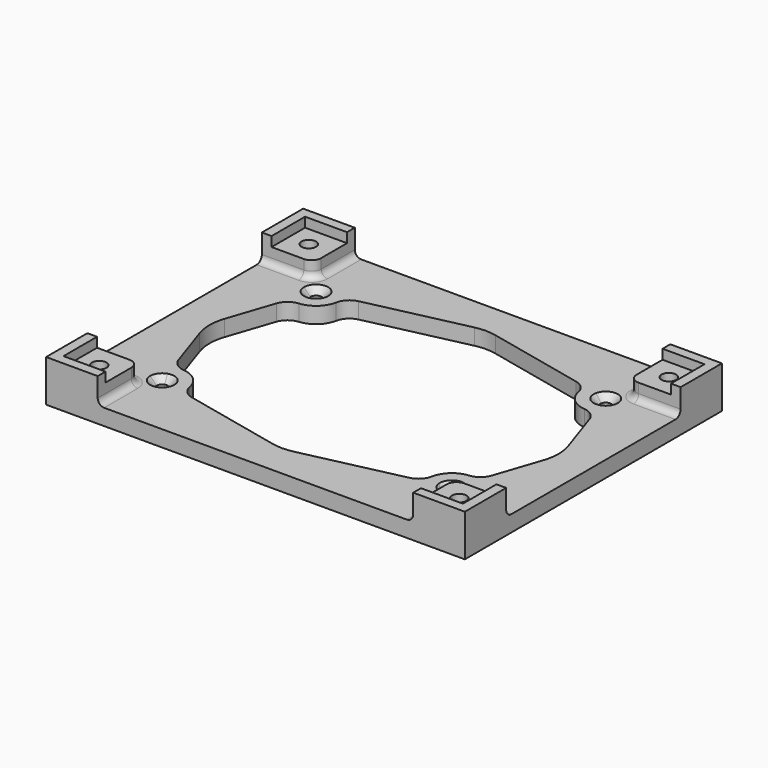
from build123d import *

# Parameters (mm, degrees)
F1_DEPTH = 5
F0_W     = 13
F0_H     = 13
F0_R     = 4
F0_R_2   = 2.25
F2_DEPTH = 10
F3_DEPTH = 13
F4_DEPTH = 6
F5_SIZE  = 2
F6_R     = 3
F7_R     = 2
F8_R     = 5
F11_R    = 15


with BuildPart() as f1:
    # F0 (on Top) → F1 (new body)
    with BuildSketch(Plane.XY):
        with BuildLine():
            ThreePointArc((43.1918518623, 30.1804338837), (45.0913645201, 31.5395055678), (46.65, 29.8))
            ThreePointArc((46.65, 29.8), (46.3207025236, 28.7781857608), (45.4567378977, 28.1409210648))
            Line((45.4567378977, 28.1409210648), (47.2860195617, 22.6896617063))
            Line((47.2860195617, 22.6896617063), (54.9, 0))
            Line((54.9, 0), (64.9, 0))
            Line((64.9, 0), (64.9, 33.8))
            Line((64.9, 33.8), (61.9, 33.8))
            Line((61.9, 33.8), (48.9, 33.8))
            Line((48.9, 33.8), (48.9, 46.8))
            Line((48.9, 46.8), (48.9, 49.8))
            Line((48.9, 49.8), (0, 49.8))
            Line((0, 49.8), (0, 39.8))
            Line((0, 39.8), (37.5793651244, 31.43043093))
            Line((37.5793651244, 31.43043093), (43.1918518623, 30.1804338837))
        make_face()
        with BuildLine():
            ThreePointArc((45.4567378977, 28.1409210648), (43.7289579343, 28.499553738), (43.1918518623, 30.1804338837))
            Line((43.1918518623, 30.1804338837), (37.5793651244, 31.43043093))
            ThreePointArc((37.5793651244, 31.43043093), (39.8812482897, 24.2266588773), (47.2860195617, 22.6896617063))
            Line((47.2860195617, 22.6896617063), (45.4567378977, 28.1409210648))
        make_face()
    extrude(amount=F1_DEPTH)

    # F0 (on Top) → F2 (join)
    with BuildSketch(Plane.XY):
        with Locations((55.4, 40.3)):
            Rectangle(F0_W, F0_H)
        with Locations((55.8, 40.6)):
            Circle(F0_R, mode=Mode.SUBTRACT)
        with Locations((55.8, 40.6)):
            Circle(F0_R)
        with Locations((55.8, 40.6)):
            Circle(F0_R_2, mode=Mode.SUBTRACT)
    extrude(amount=F2_DEPTH)

    # F0 (on Top) → F3 (join)
    with BuildSketch(Plane.XY):
        Polygon((64.9, 49.8), (48.9, 49.8), (48.9, 46.8), (61.9, 46.8), (61.9, 33.8), (64.9, 33.8), align=None)
    extrude(amount=F3_DEPTH)

    # F0 (on Top) → F4 (cut)
    with BuildSketch(Plane.XY):
        with Locations((55.8, 40.6)):
            Circle(F0_R)
        with Locations((55.8, 40.6)):
            Circle(F0_R_2, mode=Mode.SUBTRACT)
    extrude(amount=F4_DEPTH, mode=Mode.SUBTRACT)

    # F5
    f5_edges = [f1.edges().sort_by_distance(p)[0] for p in [
        (43.15, 29.8, 5),
    ]]
    chamfer(f5_edges, length=F5_SIZE)

    # F6
    f6_edges = [f1.edges().sort_by_distance(p)[0] for p in [
        (48.9, 33.8, 7.5),
    ]]
    fillet(f6_edges, radius=F6_R)

    # F7
    f7_edges = [f1.edges().sort_by_distance(p)[0] for p in [
        (58.4, 33.8, 5),
        (49.77868, 34.67868, 5),
        (48.9, 43.3, 5),
    ]]
    fillet(f7_edges, radius=F7_R)

    # F8
    f8_edges = [f1.edges().sort_by_distance(p)[0] for p in [
        (37.579365, 31.430431, 2.5),
        (47.28602, 22.689662, 2.5),
    ]]
    fillet(f8_edges, radius=F8_R)

    # F9: F1 across face


with BuildPart() as f1_1:
    add(f1.part)
    add(f1.part.mirror(Plane(origin=(0, 44.8, 2.5), x_dir=(0, -1, 0), z_dir=(-1, 0, 0))))

    # F10: F1 across face


with BuildPart() as f1_2:
    add(f1_1.part)
    add(f1_1.part.mirror(Plane(origin=(59.9, 0, 2.5), x_dir=(1, 0, 0), z_dir=(0, -1, 0))))

    # F11
    f11_edges = [f1_2.edges().sort_by_distance(p)[0] for p in [
        (0, 39.8, 2.5),
        (54.9, 0, 2.5),
        (0, -39.8, 2.5),
        (-54.9, 0, 2.5),
    ]]
    fillet(f11_edges, radius=F11_R)


solid = f1_2.part
